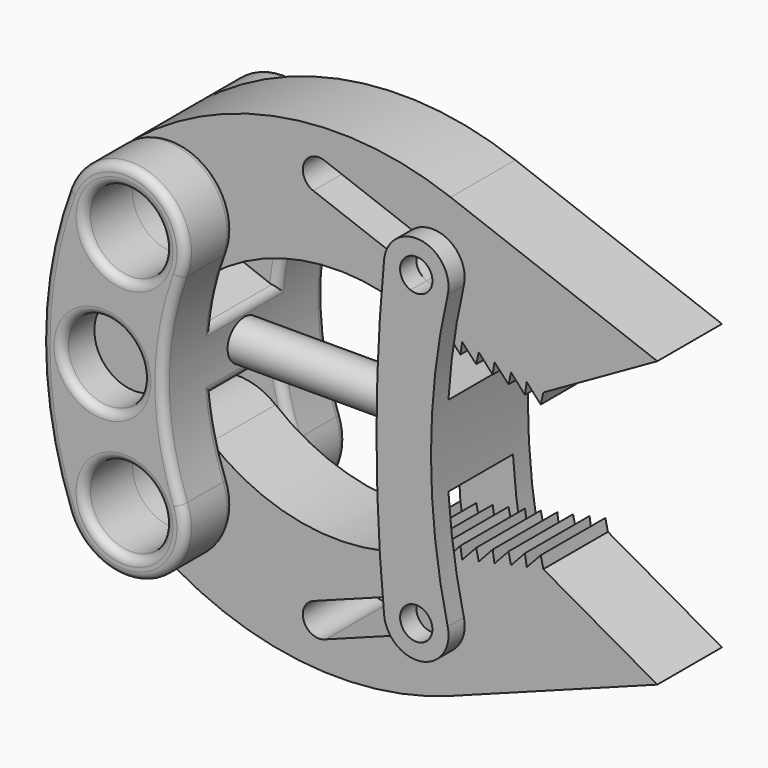
from build123d import *

# Parameters (mm, degrees)
F1_R           = 5
F2_DEPTH       = 5
F0_R           = 5
F3_DEPTH       = 12.5
F4_R           = 5
F5_DEPTH       = 25.001
F7_DEPTH       = 5
F9_R           = 2.5
F10_DEPTH      = 10.2360656985
F10_DEPTH_BACK = 60.001
F8_R           = 5
F13_DEPTH      = 5
F14_DEPTH      = 7.5
F15_DEPTH      = 32
F15_DEPTH_BACK = 10
F16_DEPTH      = 7.5
F17_DEPTH      = 5
F18_R          = 1


with BuildPart() as f2:
    # F1 (on Front) → F2 (new body, symmetric)
    with BuildSketch(Plane.XZ):
        with BuildLine():
            ThreePointArc((4.7116095582, 9.1646992048), (6.7670921261, 11.7663543551), (7.5, 15))
            ThreePointArc((7.5, 15), (3.2336456449, 21.7670921261), (-4.7116095582, 20.8353007952))
            ThreePointArc((-4.7116095582, 20.8353007952), (-5.8353007952, 10.2883904418), (4.7116095582, 9.1646992048))
        make_face()
        with Locations((0, 15)):
            Circle(F1_R, mode=Mode.SUBTRACT)
        with BuildLine():
            ThreePointArc((-4.7116095582, 20.8353007952), (3.2336456449, 21.7670921261), (7.5, 15))
            ThreePointArc((7.5, 15), (6.7670921261, 11.7663543551), (4.7116095582, 9.1646992048))
            ThreePointArc((4.7116095582, 9.1646992048), (14.7288570275, 14.0580042408), (25.8772634371, 14.1101152969))
            Line((25.8772634371, 14.1101152969), (27.8289769365, 13.6732922021))
            Line((27.8289769365, 13.6732922021), (29.8755204478, 13.2152447118))
            Line((29.8755204478, 13.2152447118), (29.8842353941, 13.2132941746))
            Line((29.8842353941, 13.2132941746), (31.8272339473, 12.778421617))
            Line((31.8272339473, 12.778421617), (33.8737774586, 12.3203741267))
            Line((33.8737774586, 12.3203741267), (33.8824924048, 12.3184235895))
            Line((33.8824924048, 12.3184235895), (35.825490958, 11.8835510319))
            Line((35.825490958, 11.8835510319), (37.8720344694, 11.4255035416))
            Line((37.8720344694, 11.4255035416), (37.8807494156, 11.4235530044))
            Line((37.8807494156, 11.4235530044), (39.8237479688, 10.9886804469))
            Line((39.8237479688, 10.9886804469), (41.8702914801, 10.5306329565))
            Line((41.8702914801, 10.5306329565), (41.8790064263, 10.5286824193))
            Line((41.8790064263, 10.5286824193), (43.8220049795, 10.0938098618))
            Line((43.8220049795, 10.0938098618), (45.8772634371, 9.6338118343))
            Line((45.8772634371, 9.6338118343), (60, 17.6338118343))
            Line((60, 17.6338118343), (34.4056996037, 27.1878953718))
            ThreePointArc((34.4056996037, 27.1878953718), (14.0050341992, 29.1964398521), (-4.7116095582, 20.8353007952))
        make_face()
        with BuildLine():
            ThreePointArc((17.3861909011, 22.3679131252), (16.2468324322, 25.0282831001), (18.9577749947, 26.0414447589))
            Line((18.9577749947, 26.0414447589), (32.8367717982, 20.8699774542))
            ThreePointArc((32.8367717982, 20.8699774542), (34.0123698575, 18.2969730456), (31.4390154577, 17.122141306))
            Line((31.4390154577, 17.122141306), (17.3861909011, 22.3679131252))
        make_face(mode=Mode.SUBTRACT)
        Polygon((27.8289769365, 13.6732922021), (25.8772634371, 14.1101152969), (27.6107883251, 12.2121614657), align=None)
        Polygon((29.8755204478, 13.2152447118), (27.8289769365, 13.6732922021), (29.5667781848, 11.7949041484), (29.882870792, 13.2071971702), align=None)
        Polygon((45.5598062278, 8.215421808), (45.8772634371, 9.6338118343), (43.8220049795, 10.0938098618), align=None)
        Polygon((29.8842353941, 13.2132941746), (29.8755204478, 13.2152447118), (29.882870792, 13.2071971702), align=None)
        Polygon((43.6038163681, 8.6326791253), (43.8220049795, 10.0938098618), (41.8790064263, 10.5286824193), (41.8776418242, 10.5225854149), align=None)
        Polygon((31.8272339473, 12.778421617), (29.8842353941, 13.2132941746), (29.882870792, 13.2071971702), (31.6090453359, 11.3172908806), align=None)
        Polygon((41.8776418242, 10.5225854149), (41.8790064263, 10.5286824193), (41.8702914801, 10.5306329565), align=None)
        Polygon((33.8737774586, 12.3203741267), (31.8272339473, 12.778421617), (33.5650351955, 10.9000335633), (33.8811278027, 12.3123265851), align=None)
        Polygon((41.8776418242, 10.5225854149), (41.8702914801, 10.5306329565), (39.8237479688, 10.9886804469), (41.561549217, 9.1102923931), align=None)
        Polygon((33.8824924048, 12.3184235895), (33.8737774586, 12.3203741267), (33.8811278027, 12.3123265851), align=None)
        Polygon((39.6055593574, 9.5275497104), (39.8237479688, 10.9886804469), (37.8807494156, 11.4235530044), (37.8793848135, 11.417456), align=None)
        Polygon((35.825490958, 11.8835510319), (33.8824924048, 12.3184235895), (33.8811278027, 12.3123265851), (35.6073023466, 10.4224202955), align=None)
        Polygon((37.8793848135, 11.417456), (37.8807494156, 11.4235530044), (37.8720344694, 11.4255035416), align=None)
        Polygon((37.8720344694, 11.4255035416), (35.825490958, 11.8835510319), (37.5632922063, 10.0051629782), (37.8793848135, 11.417456), align=None)
    extrude(amount=F2_DEPTH, both=True)


with BuildPart() as f2b:
    # F1 (on Front) → F2, piece 2 (new body, symmetric)
    with BuildSketch(Plane.XZ):
        with BuildLine():
            ThreePointArc((-4.7116095582, -20.8353007952), (3.2336456449, -21.7670921261), (7.5, -15))
            ThreePointArc((7.5, -15), (6.7670921261, -11.7663543551), (4.7116095582, -9.1646992048))
            ThreePointArc((4.7116095582, -9.1646992048), (-5.8353007952, -10.2883904418), (-4.7116095582, -20.8353007952))
        make_face()
        with Locations((0, -15)):
            Circle(F1_R, mode=Mode.SUBTRACT)
        with BuildLine():
            ThreePointArc((4.7116095582, -9.1646992048), (6.7670921261, -11.7663543551), (7.5, -15))
            ThreePointArc((7.5, -15), (3.2336456449, -21.7670921261), (-4.7116095582, -20.8353007952))
            ThreePointArc((-4.7116095582, -20.8353007952), (14.0050341992, -29.1964398521), (34.4056996037, -27.1878953718))
            Line((34.4056996037, -27.1878953718), (60, -17.6338118343))
            Line((60, -17.6338118343), (45.8772634371, -9.6338118343))
            Line((45.8772634371, -9.6338118343), (43.8220049795, -10.0938098618))
            Line((43.8220049795, -10.0938098618), (41.8790064263, -10.5286824193))
            Line((41.8790064263, -10.5286824193), (41.8702914801, -10.5306329565))
            Line((41.8702914801, -10.5306329565), (39.8237479688, -10.9886804469))
            Line((39.8237479688, -10.9886804469), (37.8807494156, -11.4235530044))
            Line((37.8807494156, -11.4235530044), (37.8720344694, -11.4255035416))
            Line((37.8720344694, -11.4255035416), (35.825490958, -11.8835510319))
            Line((35.825490958, -11.8835510319), (33.8824924048, -12.3184235895))
            Line((33.8824924048, -12.3184235895), (33.8737774586, -12.3203741267))
            Line((33.8737774586, -12.3203741267), (31.8272339473, -12.778421617))
            Line((31.8272339473, -12.778421617), (29.8842353941, -13.2132941746))
            Line((29.8842353941, -13.2132941746), (29.8755204478, -13.2152447118))
            Line((29.8755204478, -13.2152447118), (27.8289769365, -13.6732922021))
            Line((27.8289769365, -13.6732922021), (25.8772634371, -14.1101152969))
            ThreePointArc((25.8772634371, -14.1101152969), (14.7288570275, -14.0580042408), (4.7116095582, -9.1646992048))
        make_face()
        with BuildLine():
            Line((32.8367717982, -20.8699774542), (18.9577749947, -26.0414447589))
            ThreePointArc((18.9577749947, -26.0414447589), (16.2468324322, -25.0282831001), (17.3861909011, -22.3679131252))
            Line((17.3861909011, -22.3679131252), (31.4390154577, -17.122141306))
            ThreePointArc((31.4390154577, -17.122141306), (34.0123698575, -18.2969730456), (32.8367717982, -20.8699774542))
        make_face(mode=Mode.SUBTRACT)
        Polygon((27.6107883251, -12.2121614657), (25.8772634371, -14.1101152969), (27.8289769365, -13.6732922021), align=None)
        Polygon((29.5667781848, -11.7949041484), (27.8289769365, -13.6732922021), (29.8755204478, -13.2152447118), (29.882870792, -13.2071971702), align=None)
        Polygon((29.882870792, -13.2071971702), (29.8755204478, -13.2152447118), (29.8842353941, -13.2132941746), align=None)
        Polygon((43.8220049795, -10.0938098618), (45.8772634371, -9.6338118343), (45.5598062278, -8.215421808), align=None)
        Polygon((29.882870792, -13.2071971702), (29.8842353941, -13.2132941746), (31.8272339473, -12.778421617), (31.6090453359, -11.3172908806), align=None)
        Polygon((41.8790064263, -10.5286824193), (43.8220049795, -10.0938098618), (43.6038163681, -8.6326791253), (41.8776418242, -10.5225854149), align=None)
        Polygon((33.5650351955, -10.9000335633), (31.8272339473, -12.778421617), (33.8737774586, -12.3203741267), (33.8811278027, -12.3123265851), align=None)
        Polygon((41.8702914801, -10.5306329565), (41.8790064263, -10.5286824193), (41.8776418242, -10.5225854149), align=None)
        Polygon((33.8811278027, -12.3123265851), (33.8737774586, -12.3203741267), (33.8824924048, -12.3184235895), align=None)
        Polygon((39.8237479688, -10.9886804469), (41.8702914801, -10.5306329565), (41.8776418242, -10.5225854149), (41.561549217, -9.1102923931), align=None)
        Polygon((33.8811278027, -12.3123265851), (33.8824924048, -12.3184235895), (35.825490958, -11.8835510319), (35.6073023466, -10.4224202955), align=None)
        Polygon((37.8807494156, -11.4235530044), (39.8237479688, -10.9886804469), (39.6055593574, -9.5275497104), (37.8793848135, -11.417456), align=None)
        Polygon((37.5632922063, -10.0051629782), (35.825490958, -11.8835510319), (37.8720344694, -11.4255035416), (37.8793848135, -11.417456), align=None)
        Polygon((37.8720344694, -11.4255035416), (37.8807494156, -11.4235530044), (37.8793848135, -11.417456), align=None)
    extrude(amount=F2_DEPTH, both=True)


with BuildPart() as f3:
    # F0 (on Front) → F3 (new body, symmetric)
    with BuildSketch(Plane.XZ):
        with BuildLine():
            ThreePointArc((7.0173413473, -12.3529411765), (4.7649343015, 0), (7.0173413473, 12.3529411765))
            ThreePointArc((7.0173413473, 12.3529411765), (2.6470588235, 22.0173413473), (-7.0173413473, 17.6470588235))
            ThreePointArc((-7.0173413473, 17.6470588235), (-10.2350656985, 0), (-7.0173413473, -17.6470588235))
            ThreePointArc((-7.0173413473, -17.6470588235), (2.6470588235, -22.0173413473), (7.0173413473, -12.3529411765))
        make_face()
        with Locations((0, -15)):
            Circle(F0_R, mode=Mode.SUBTRACT)
        with Locations((0, 15)):
            Circle(F0_R, mode=Mode.SUBTRACT)
    extrude(amount=F3_DEPTH, both=True)

    # F4 (on face) → F5 (cut, through all)
    with BuildSketch(Plane.XZ.offset(12.5)):
        with Locations((-2.7350656985, 0)):
            Circle(F4_R)
    extrude(amount=-F5_DEPTH, mode=Mode.SUBTRACT)

    # F6 (on Front) → F7 (cut, symmetric)
    with BuildSketch(Plane.XZ):
        with BuildLine():
            Line((-9.4296987911, 8.938012916), (4.942060921, 3.5167441658))
            ThreePointArc((4.942060921, 3.5167441658), (5.692048093, 8.0024012288), (7.0173413473, 12.3529411765))
            ThreePointArc((7.0173413473, 12.3529411765), (2.6470588235, 22.0173413473), (-7.0173413473, 17.6470588235))
            ThreePointArc((-7.0173413473, 17.6470588235), (-8.4206820487, 13.3471486452), (-9.4296987911, 8.938012916))
        make_face()
        with BuildLine():
            ThreePointArc((7.0173413473, -12.3529411765), (5.692048093, -8.0024012288), (4.942060921, -3.5167441658))
            Line((4.942060921, -3.5167441658), (-9.4296987911, -8.938012916))
            ThreePointArc((-9.4296987911, -8.938012916), (-8.4206820487, -13.3471486452), (-7.0173413473, -17.6470588235))
            ThreePointArc((-7.0173413473, -17.6470588235), (2.6470588235, -22.0173413473), (7.0173413473, -12.3529411765))
        make_face()
    extrude(amount=F7_DEPTH, both=True, mode=Mode.SUBTRACT)

    # F9 (on Right) → F10 (cut, two sides)
    with BuildSketch(Plane.YZ) as f10_sk:
        Circle(F9_R)
    extrude(amount=-F10_DEPTH, mode=Mode.SUBTRACT)
    extrude(f10_sk.sketch, amount=F10_DEPTH_BACK, mode=Mode.SUBTRACT)

    # F8 (on Front) → F13 (join, symmetric)
    with BuildSketch(Plane.XZ):
        with Locations((-2.7350656985, 0)):
            Circle(F8_R)
    extrude(amount=F13_DEPTH, both=True)

    # F8 (on Front) → F14 (join, symmetric)
    with BuildSketch(Plane.XZ):
        with Locations((-2.7350656985, 0)):
            Circle(F8_R)
    extrude(amount=F14_DEPTH, both=True)

    # F18
    f18_edges = [f3.edges().sort_by_distance(p)[0] for p in [
        (4.764934, -12.5, 0),
        (2.647059, -12.5, 22.017341),
        (-10.235066, 12.5, 0),
        (2.647059, 12.5, 22.017341),
        (4.764934, 12.5, 0),
        (2.647059, 12.5, -22.017341),
        (-10.235066, -12.5, 0),
        (2.647059, -12.5, -22.017341),
        (-5, -12.5, -15),
        (-7.735066, -12.5, 0),
        (-5, -12.5, 15),
        (5.692048, -5, -8.002401),
        (4.942061, 0, -3.516744),
        (4.942061, 0, 3.516744),
        (5.692048, 5, 8.002401),
        (5.692048, 5, -8.002401),
        (5.692048, -5, 8.002401),
        (-8.420682, 5, 13.347149),
        (-8.420682, -5, 13.347149),
        (-8.420682, -5, -13.347149),
        (-8.420682, 5, -13.347149),
    ]]
    fillet(f18_edges, radius=F18_R)


with BuildPart() as f15:
    # F9 (on Right) → F15 (new body, two sides)
    with BuildSketch(Plane.YZ) as f15_sk:
        Circle(F9_R)
    extrude(amount=F15_DEPTH)
    extrude(f15_sk.sketch, amount=-F15_DEPTH_BACK)

    # F11 (on Front) → F16 (join, symmetric)
    with BuildSketch(Plane.XZ):
        with BuildLine():
            ThreePointArc((36.0348299347, -18.0912869018), (33.9623946229, 0), (36.0348299347, 18.0912869018))
            ThreePointArc((36.0348299347, 18.0912869018), (32.7859585158, 22.9430952124), (28.1572820688, 19.3835216805))
            ThreePointArc((28.1572820688, 19.3835216805), (27.2157636446, 0), (28.1572820688, -19.3835216805))
            ThreePointArc((28.1572820688, -19.3835216805), (32.7859585158, -22.9430952124), (36.0348299347, -18.0912869018))
        make_face()
        with BuildLine():
            ThreePointArc((32.8367717982, -20.8699774542), (30.2645335431, -19.6947294481), (31.4390154577, -17.122141306))
            ThreePointArc((31.4390154577, -17.122141306), (33.2788743226, -17.3528551292), (34.1384517003, -18.9958512469))
            ThreePointArc((34.1384517003, -18.9958512469), (33.7811081153, -20.1367631199), (32.8367717982, -20.8699774542))
        make_face(mode=Mode.SUBTRACT)
        with BuildLine():
            ThreePointArc((34.1384517003, 18.9958512469), (33.2788743226, 17.3528551292), (31.4390154577, 17.122141306))
            ThreePointArc((31.4390154577, 17.122141306), (30.2645335431, 19.6947294481), (32.8367717982, 20.8699774542))
            ThreePointArc((32.8367717982, 20.8699774542), (33.7811081153, 20.1367631199), (34.1384517003, 18.9958512469))
        make_face(mode=Mode.SUBTRACT)
    extrude(amount=F16_DEPTH, both=True)

    # F12 (on Front) → F17 (cut, symmetric)
    with BuildSketch(Plane.XZ):
        with BuildLine():
            ThreePointArc((28.1572820688, 19.3835216805), (27.5881908908, 12.1996801778), (27.2782734133, 5))
            Line((27.2782734133, 5), (34.1187975096, 5))
            ThreePointArc((34.1187975096, 5), (34.8057125156, 11.5853216511), (36.0348299347, 18.0912869018))
            ThreePointArc((36.0348299347, 18.0912869018), (32.7859585158, 22.9430952124), (28.1572820688, 19.3835216805))
        make_face()
        with BuildLine():
            ThreePointArc((28.1572820688, -19.3835216805), (32.7859585158, -22.9430952124), (36.0348299347, -18.0912869018))
            ThreePointArc((36.0348299347, -18.0912869018), (34.8057125156, -11.5853216511), (34.1187975096, -5))
            Line((34.1187975096, -5), (27.2782734133, -5))
            ThreePointArc((27.2782734133, -5), (27.5881908908, -12.1996801778), (28.1572820688, -19.3835216805))
        make_face()
    extrude(amount=F17_DEPTH, both=True, mode=Mode.SUBTRACT)


solid = Compound([f2.part, f2b.part, f3.part, f15.part])
